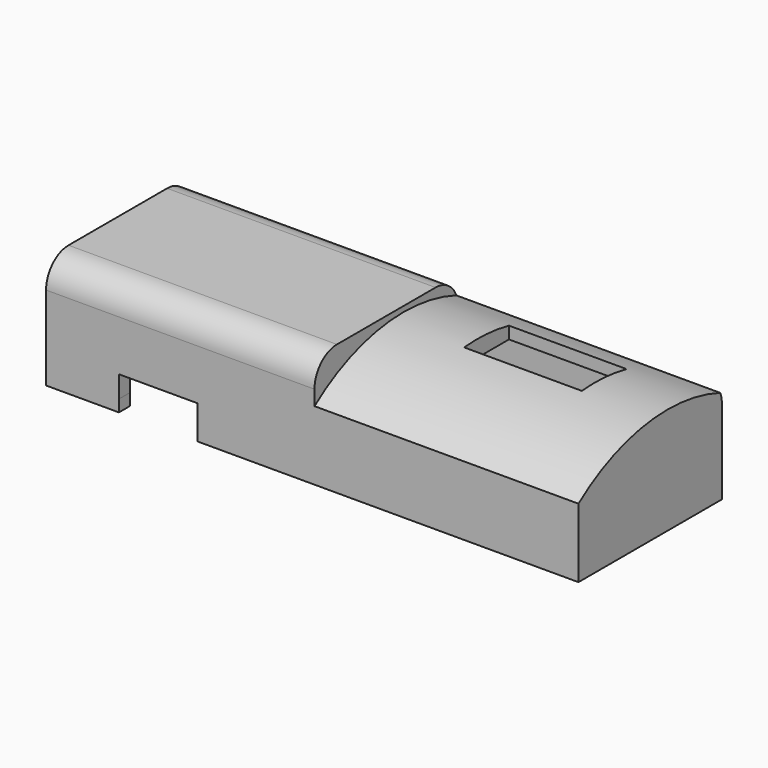
from build123d import *

# Parameters (mm, degrees)
F0_W        = 95
F0_H        = 32
F1_DEPTH    = 20
F3_R        = 5
F4_R        = 5
F6_DEPTH    = 25
F7_DEPTH    = 47.1
F8_T        = 2.5
F8_T3_DEPTH = 23.9149246247
F8_T5_DEPTH = 23.2696171533
F8_T8_ANGLE = 58.1590270575
F9_W        = 21
F9_H        = 10
F10_DEPTH   = 16.1
F13_DEPTH   = 25


# Not quite as in the source:
# - a shell that OpenCascade refuses in one call is made with other operations: the cavity is built on its own and cut out


with BuildPart() as f1:
    # F0 (on Top) → F1 (new body)
    with BuildSketch(Plane.XY):
        with Locations((66.9030988216, -21.9037037492)):
            Rectangle(F0_W, F0_H)
    extrude(amount=F1_DEPTH)

    # F3
    f3_edges = [f1.edges().sort_by_distance(p)[0] for p in [
        (66.903099, -37.903704, 20),
    ]]
    fillet(f3_edges, radius=F3_R)

    # F4
    f4_edges = [f1.edges().sort_by_distance(p)[0] for p in [
        (66.903099, -5.903704, 20),
    ]]
    fillet(f4_edges, radius=F4_R)

    # F5 (on face) → F6 (cut)
    with BuildSketch(Plane.XY.offset(20)):
        Polygon((101.4030988216, -20.6582732499), (101.4030988216, -10.9037037492), (80.4030988216, -10.9037037492), (80.4030988216, -20.9037037492), (101.4030988216, -20.9037037492), align=None)
    extrude(amount=-F6_DEPTH, mode=Mode.SUBTRACT)

    # F2 (on face) → F7 (cut)
    with BuildSketch(Plane.YZ.offset(114.4030988216)):
        with BuildLine():
            ThreePointArc((-37.9037037492, 12.3313413933), (-22.4823614594, 18.7362249856), (-5.9037037492, 16.7391169816))
            Line((-5.9037037492, 16.7391169816), (-5.9037037492, 20))
            Line((-5.9037037492, 20), (-37.9037037492, 20))
            Line((-37.9037037492, 20), (-37.9037037492, 12.3313413933))
        make_face()
    extrude(amount=-F7_DEPTH, mode=Mode.SUBTRACT)

    # F8: shell of thickness 2.5, made by hand


with BuildPart() as f8_core1:
    # F8_t2: copy of F1
    add(f1.part)

    # the walls: a layer under each face that stays
    f8_faces = [f8_core1.faces().sort_by_distance(p)[0] for p in [
        (19.4030988216, -21.9037037492, 10),
        (43.3530988216, -21.9037037492, 20),
        (66.9030988216, -7.3681698432, 18.5355339059),
        (43.3530988216, -36.4392376551, 18.5355339059),
        (66.9030988216, -5.9037037492, 7.5),
        (66.9030988216, -37.9037037492, 7.5),
        (67.3030988216, -32.6316572711, 16.1656706966),
        (90.8530988216, -22.6776915616, 18.7087222914),
        (114.4030988216, -21.9037037492, 9.5218727657),
        (80.4030988216, -15.9037037492, 9.5218727657),
        (90.9030988216, -20.9037037492, 9.4574623123),
        (101.4030988216, -15.9037037492, 9.5218727657),
        (90.9030988216, -10.9037037492, 9.1348085767),
    ]]
    thicken(f8_faces, amount=-F8_T, mode=Mode.SUBTRACT)

    # F8_s4 → F8_t3 (cut)
    with BuildSketch(Plane.XY.offset(-2.5)):
        Polygon((80.4280988216, -20.8787037492), (77.9030988216, -20.9037037492), (77.9030988216, -23.4037037492), (80.4030988216, -23.4037037492), align=None)
        Polygon((101.3780988216, -20.8787037492), (101.4030988216, -23.4037037492), (103.9030988216, -23.4037037492), (103.9030988216, -20.9037037492), align=None)
    extrude(amount=F8_T3_DEPTH, mode=Mode.SUBTRACT)

    # F8_s6 → F8_t5 (cut)
    with BuildSketch(Plane.XY.offset(-2.5)):
        Polygon((80.4280988216, -10.9287037492), (77.9030988216, -10.9037037492), (77.9030988216, -8.4037037492), (80.4030988216, -8.4037037492), align=None)
        Polygon((101.3780988216, -10.9287037492), (103.9030988216, -10.9037037492), (103.9030988216, -8.4037037492), (101.4030988216, -8.4037037492), align=None)
    extrude(amount=F8_T5_DEPTH, mode=Mode.SUBTRACT)

    # F8_s7 → F8_t8 (revolve, cut)
    with BuildSketch(Plane(origin=(0, -18.0639523955, -13.7441213447), x_dir=(1, 0, 0), z_dir=(0, -0.7958327334, -0.6055165237))):
        Polygon((67.3280988216, 32.7900040558), (64.8030988216, 32.7650040558), (64.8030988216, 30.2650040558), (67.3030988216, 30.2650040558), align=None)
    revolve(axis=Axis((67.3030988216, -17.9961461515, -13.8332393562), (-1, 0, 0)), revolution_arc=F8_T8_ANGLE, mode=Mode.SUBTRACT)


with BuildPart() as f1_1:
    add(f1.part)

    # what is left inside the walls is the cavity
    f8_cavity = [f8_core1.part.solids().sort_by_distance(p)[0] for p in [
        (66.903099, -26.403704, 0.025),
    ]]
    add(f8_cavity, mode=Mode.SUBTRACT)

    # F9 (on face) → F10 (cut)
    with BuildSketch(Plane(origin=(0, 0, 0), x_dir=(1, 0, 0), z_dir=(0, 0, -1))):
        Polygon((77.9030988216, 10.9037037492), (77.9030988216, 8.4037037492), (103.9030988216, 8.4037037492), (103.9030988216, 10.9037037492), (103.9030988216, 20.9037037492), (103.9030988216, 23.4037037492), (77.9030988216, 23.4037037492), (77.9030988216, 20.9037037492), align=None)
        with Locations((90.9030988216, 15.9037037492)):
            Rectangle(F9_W, F9_H, mode=Mode.SUBTRACT)
    extrude(amount=-F10_DEPTH, mode=Mode.SUBTRACT)

    # F12 (on face) → F13 (cut)
    with BuildSketch(Plane.XZ.offset(37.9037037492)):
        Polygon((46.4005000293, 6), (32.4030988216, 6), (32.4030988216, 2.1138605662), (32.4005000293, 2.1138605662), (32.4005000293, 0), (46.4005000293, 0), align=None)
    extrude(amount=-F13_DEPTH, mode=Mode.SUBTRACT)


solid = f1_1.part
